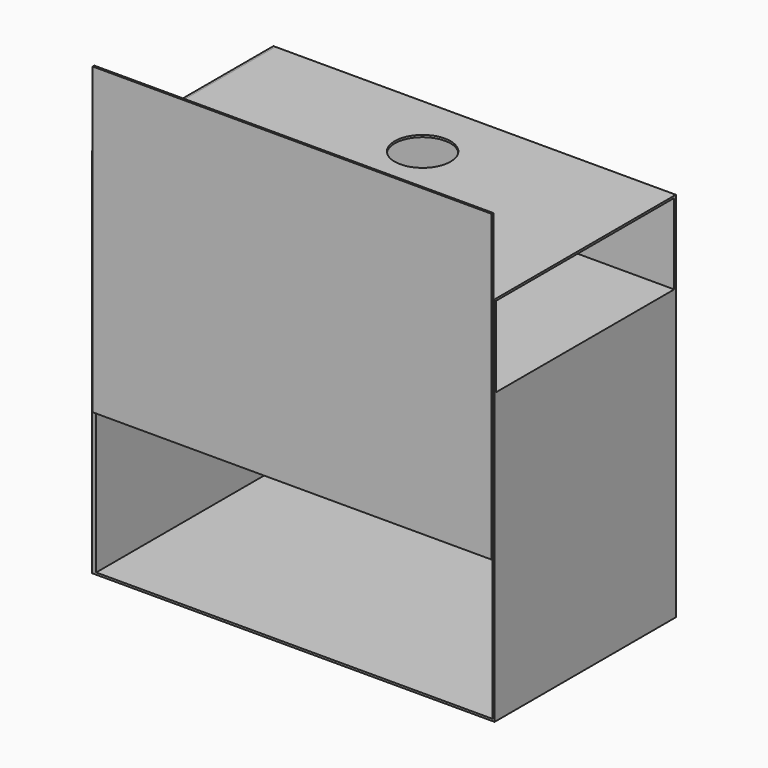
from build123d import *

# Parameters (mm, degrees)
F0_W      = 65.8
F0_H      = 23.8
F1_DEPTH  = 118.4
F2_DEPTH  = 0.6
F3_W      = 65.8
F3_H      = 23.8
F2_FACE_W = 67
F2_FACE_H = 110
F4_DEPTH  = 0.6
F7_DEPTH  = 1
F8_W      = 118
F8_H      = 0.6
F9_DEPTH  = 90
F10_DEPTH = 25


# Not quite as in the source:
# - a feature names something its author has since deleted; it is built from what else it names


with BuildPart() as f1:
    # F0 (on Right) → F1 (new body)
    with BuildSketch(Plane.YZ):
        Polygon((5.5, 42.5), (4.6354143734, 42.5), (10.5434493031, 36.8055236056), (22.9, 24.8956268129), (22.9, -12.5), (23.5, -12.5), (23.5, 25.1506484271), align=None)
        Polygon((-33.5, -42.5), (33.5, -42.5), (33.5, 42.5), (33.5, 67.5), (-33.5, 67.5), (-33.5, 43.1), (-33.5, 42.5), (4.6354143734, 42.5), (5.5, 42.5), (32.9, 42.5), (32.9, -41.9), (-32.9, -41.9), (-33.5, -41.9), align=None)
        with Locations((0, 55)):
            Rectangle(F0_W, F0_H, mode=Mode.SUBTRACT)
    extrude(amount=F1_DEPTH)

    # F3 (on face) + F0 (on Right) + F2_face (on face) → F4 (join)
    with BuildSketch(Plane.YZ.offset(118.4)):
        Polygon((-33.5, -42.5), (33.5, -42.5), (33.5, 42.5), (33.5, 67.5), (-33.5, 67.5), (-33.5, 42.5), (4.6354143734, 42.5), (22.9, 24.8956268129), (22.9, -12.5), (23.5, -12.5), (23.5, 25.1506484271), (5.5, 42.5), (32.9, 42.5), (32.9, -41.9), (-33.5, -41.9), align=None)
        with Locations((0, 55)):
            Rectangle(F3_W, F3_H, mode=Mode.SUBTRACT)
        Polygon((-33.5, 42.5), (-33.5, -41.9), (32.9, -41.9), (32.9, 42.5), (5.5, 42.5), (23.5, 25.1506484271), (23.5, -12.5), (22.9, -12.5), (22.9, 24.8956268129), (4.6354143734, 42.5), align=None)
    with BuildSketch(Plane.YZ):
        Polygon((-33.5, -42.5), (33.5, -42.5), (33.5, 42.5), (33.5, 67.5), (-33.5, 67.5), (-33.5, 43.1), (-33.5, 42.5), (4.6354143734, 42.5), (5.5, 42.5), (32.9, 42.5), (32.9, -41.9), (-32.9, -41.9), (-33.5, -41.9), align=None)
        with Locations((0, 55)):
            Rectangle(F0_W, F0_H, mode=Mode.SUBTRACT)
    with BuildSketch(Plane(origin=(0.6, 0, 12.5), x_dir=(0, 1, 0), z_dir=(1, 0, 0))):
        Rectangle(F2_FACE_W, F2_FACE_H)
    extrude(amount=F4_DEPTH)

    # F6 (on face) → F7 (cut)
    with BuildSketch(Plane(origin=(0, 23.4680218875, 24.3481372891), x_dir=(1, 0, 0), z_dir=(0, -0.6939740629, -0.72))):
        with BuildLine():
            Line((10.3, 20.156399325), (109.3, 20.156399325))
            ThreePointArc((109.3, 20.156399325), (109.6535533906, 20.3028459345), (109.8, 20.656399325))
            ThreePointArc((109.8, 20.656399325), (109.6535533906, 21.0099527156), (109.3, 21.156399325))
            Line((109.3, 21.156399325), (10.3, 21.156399325))
            ThreePointArc((10.3, 21.156399325), (9.9464466094, 21.0099527156), (9.8, 20.656399325))
            ThreePointArc((9.8, 20.656399325), (9.9464466094, 20.3028459345), (10.3, 20.156399325))
        make_face()
    extrude(amount=-F7_DEPTH, mode=Mode.SUBTRACT)

    # F5 (on face) → F10 (cut)
    with BuildSketch(Plane.XY.offset(67.5)):
        with BuildLine():
            ThreePointArc((51.55, 13.8999999701), (59.8000000075, 5.649999985), (68.05, 13.899999985))
            Line((68.05, 13.8999999701), (51.55, 13.8999999701))
        make_face()
        with BuildLine():
            Line((51.55, 13.8999999701), (68.05, 13.8999999701))
            ThreePointArc((68.05, 13.899999985), (59.7999999925, 22.149999985), (51.55, 13.8999999701))
        make_face()
    extrude(amount=-F10_DEPTH, mode=Mode.SUBTRACT)


with BuildPart() as f2:
    # F0 (on Right) → F2 (new body)
    with BuildSketch(Plane.YZ):
        Polygon((-33.5, 42.5), (-33.5, -41.9), (-32.9, -41.9), (32.9, -41.9), (32.9, 42.5), (5.5, 42.5), (23.5, 25.1506484271), (23.5, -12.5), (22.9, -12.5), (22.9, 24.8956268129), (10.5434493031, 36.8055236056), (4.6354143734, 42.5), align=None)
        Polygon((-33.5, -42.5), (33.5, -42.5), (33.5, 42.5), (33.5, 67.5), (-33.5, 67.5), (-33.5, 43.1), (-33.5, 42.5), (4.6354143734, 42.5), (5.5, 42.5), (32.9, 42.5), (32.9, -41.9), (-32.9, -41.9), (-33.5, -41.9), align=None)
        with Locations((0, 55)):
            Rectangle(F0_W, F0_H, mode=Mode.SUBTRACT)
        with Locations((0, 55)):
            Rectangle(F0_W, F0_H)
        Polygon((5.5, 42.5), (4.6354143734, 42.5), (10.5434493031, 36.8055236056), (22.9, 24.8956268129), (22.9, -12.5), (23.5, -12.5), (23.5, 25.1506484271), align=None)
    extrude(amount=F2_DEPTH)


with BuildPart() as f9:
    # F8 (on Top) → F9 (new body)
    with BuildSketch(Plane.XY):
        with Locations((59.8, -34)):
            Rectangle(F8_W, F8_H)
    extrude(amount=F9_DEPTH)


solid = Compound([f1.part, f2.part, f9.part])
